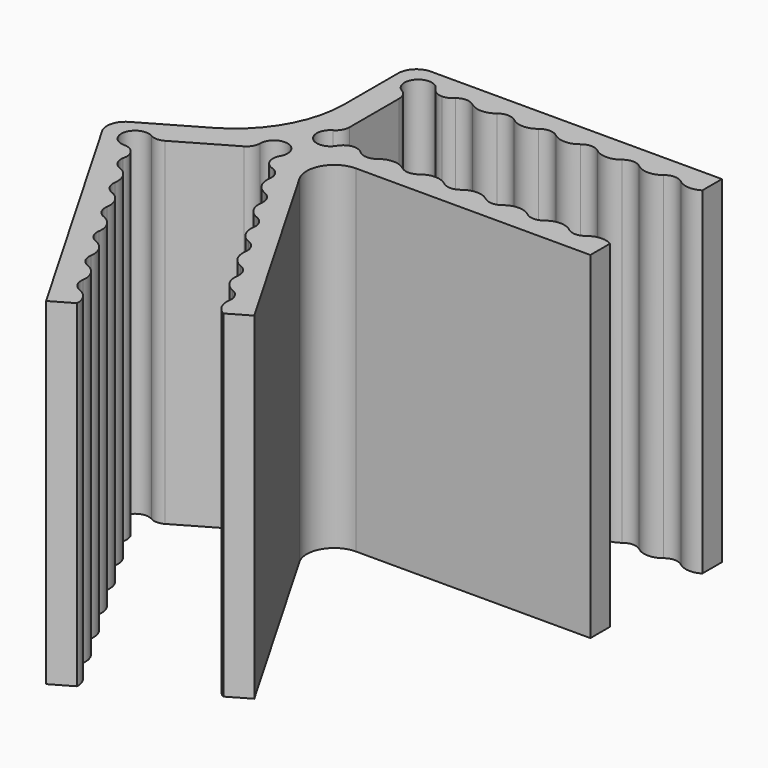
from build123d import *

# Parameters (mm, degrees)
F2_DEPTH  = 24
F3_R      = 1.95
F4_R      = 1.3
F5_R      = 7.8
F6_R      = 0.975
F7_DEPTH  = 24.001
F8_R      = 0.975
F10_DEPTH = 24.001


# Not quite as in the source:
# - a pattern or mirror of a feature is missing from the dataset's text; its kind, count and spacing are read off the source's solid


with BuildPart() as f2:
    # F1 (on Top) → F2 (new body)
    with BuildSketch(Plane.XY):
        Polygon((-38.45, 35.7249907476), (-58.5, 35.7249907476), (-58.5, 43.5249907476), (-38.45, 43.5249907476), (-38.45, 45.4749907476), (-60.45, 45.4749907476), (-60.45, 34.9008237725), (-69.6074972243, 29.613740285), (-58.6074972243, 10.5611814017), (-56.9187476869, 11.5361814017), (-66.9437476869, 28.8999907476), (-60.1887495374, 32.7999907476), (-50.1637495374, 15.4361814017), (-48.475, 16.4111814017), (-58.5, 33.7749907476), (-38.45, 33.7749907476), align=None)
    extrude(amount=F2_DEPTH)

    # F3
    f3_edges = [f2.edges().sort_by_distance(p)[0] for p in [
        (-58.5, 33.774991, 12),
    ]]
    fillet(f3_edges, radius=F3_R)

    # F4
    f4_edges = [f2.edges().sort_by_distance(p)[0] for p in [
        (-60.45, 45.474991, 12),
        (-69.607497, 29.61374, 12),
    ]]
    fillet(f4_edges, radius=F4_R)

    # F5
    f5_edges = [f2.edges().sort_by_distance(p)[0] for p in [
        (-60.45, 34.900824, 12),
    ]]
    fillet(f5_edges, radius=F5_R)

    # F6 (on face) → F7 (cut, through all)
    with BuildSketch(Plane.XY.offset(24)):
        with Locations((-58.5, 43.5249907476)):
            Circle(F6_R)
        with Locations((-58.5, 35.7249907476)):
            Circle(F6_R)
        with Locations((-60.1887495374, 32.7999907476)):
            Circle(F6_R)
        with Locations((-66.9437476869, 28.8999907476)):
            Circle(F6_R)
    extrude(amount=-F7_DEPTH, mode=Mode.SUBTRACT)

    # F8
    f8_edges = [f2.edges().sort_by_distance(p)[0] for p in [
        (-57.525, 43.524991, 12),
        (-58.5, 42.549991, 12),
        (-58.5, 36.699991, 12),
        (-61.033124, 32.312491, 12),
        (-66.099373, 29.387491, 12),
        (-66.456248, 28.055616, 12),
        (-59.70125, 31.955616, 12),
        (-57.525, 35.724991, 12),
    ]]
    fillet(f8_edges, radius=F8_R)

    # F9 (on face) → F10 (cut, through all)
    with BuildSketch(Plane.XY.offset(24)):
        with BuildLine():
            ThreePointArc((-56.8112504626, 35.7249907476), (-56.4247739612, 35.6451225333), (-56.1016147685, 35.4186028785))
            ThreePointArc((-56.1016147685, 35.4186028785), (-55.4926155069, 35.2050126889), (-54.8836162453, 35.4186028785))
            ThreePointArc((-54.8836162453, 35.4186028785), (-54.0100274986, 35.7249907476), (-53.1364387518, 35.4186028785))
            ThreePointArc((-53.1364387518, 35.4186028785), (-52.5274394902, 35.2050126889), (-51.9184402287, 35.4186028785))
            ThreePointArc((-51.9184402287, 35.4186028785), (-51.0448514819, 35.7249907476), (-50.1712627351, 35.4186028785))
            ThreePointArc((-50.1712627351, 35.4186028785), (-49.5622634735, 35.2050126889), (-48.953264212, 35.4186028785))
            ThreePointArc((-48.953264212, 35.4186028785), (-48.0796754652, 35.7249907476), (-47.2060867184, 35.4186028785))
            ThreePointArc((-47.2060867184, 35.4186028785), (-46.5970874569, 35.2050126889), (-45.9880881953, 35.4186028785))
            ThreePointArc((-45.9880881953, 35.4186028785), (-45.1144994485, 35.7249907475), (-44.2409107018, 35.4186028784))
            ThreePointArc((-44.2409107018, 35.4186028784), (-43.6319114402, 35.2050126889), (-43.0229121786, 35.4186028784))
            ThreePointArc((-43.0229121786, 35.4186028784), (-42.1493234318, 35.7249907475), (-41.2757346851, 35.4186028784))
            ThreePointArc((-41.2757346851, 35.4186028784), (-40.6667354235, 35.2050126888), (-40.0577361619, 35.4186028784))
            ThreePointArc((-40.0577361619, 35.4186028784), (-39.1841474152, 35.7249907475), (-38.3105586684, 35.4186028784))
            Line((-38.3105586684, 35.4186028784), (-38.3105586684, 43.8313786168))
            ThreePointArc((-38.3105586684, 43.8313786168), (-39.1841474152, 43.5249907477), (-40.0577361619, 43.8313786168))
            ThreePointArc((-40.0577361619, 43.8313786168), (-40.6667354235, 44.0449688064), (-41.2757346851, 43.8313786168))
            ThreePointArc((-41.2757346851, 43.8313786168), (-42.1493234318, 43.5249907477), (-43.0229121786, 43.8313786168))
            ThreePointArc((-43.0229121786, 43.8313786168), (-43.6319114402, 44.0449688063), (-44.2409107018, 43.8313786168))
            ThreePointArc((-44.2409107018, 43.8313786168), (-45.1144994485, 43.5249907476), (-45.9880881953, 43.8313786167))
            ThreePointArc((-45.9880881953, 43.8313786167), (-46.5970874569, 44.0449688063), (-47.2060867184, 43.8313786167))
            ThreePointArc((-47.2060867184, 43.8313786167), (-48.0796754652, 43.5249907476), (-48.953264212, 43.8313786167))
            ThreePointArc((-48.953264212, 43.8313786167), (-49.5622634735, 44.0449688063), (-50.1712627351, 43.8313786167))
            ThreePointArc((-50.1712627351, 43.8313786167), (-51.0448514819, 43.5249907476), (-51.9184402287, 43.8313786167))
            ThreePointArc((-51.9184402287, 43.8313786167), (-52.5274394902, 44.0449688063), (-53.1364387518, 43.8313786167))
            ThreePointArc((-53.1364387518, 43.8313786167), (-54.0100274986, 43.5249907476), (-54.8836162453, 43.8313786167))
            ThreePointArc((-54.8836162453, 43.8313786167), (-55.4926155069, 44.0449688063), (-56.1016147685, 43.8313786167))
            ThreePointArc((-56.1016147685, 43.8313786167), (-56.4247739612, 43.6048589619), (-56.8112504626, 43.5249907476))
            Line((-56.8112504626, 43.5249907476), (-56.8112504626, 35.7249907476))
        make_face()
    f10 = extrude(amount=-F10_DEPTH, mode=Mode.SUBTRACT)

    # F10_copies: F10 across plane
    add(f10.mirror(Plane(origin=(0, 0, 0), x_dir=(-0.8660254031, 0.5000000012, 0), z_dir=(-0.5000000012, -0.8660254031, 0))), mode=Mode.SUBTRACT)


solid = f2.part
